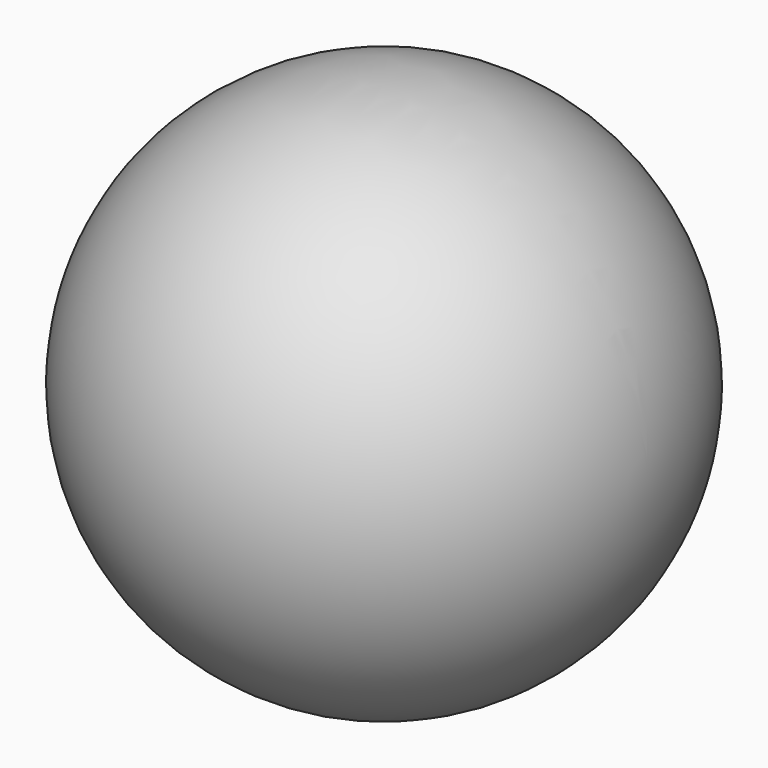
from build123d import *

# Parameters (mm, degrees)
F0_R = 11.165731945


# Not quite as in the source:
# - a feature of the source that left no trace in its solid (it failed there, or was rolled back) is left out


with BuildPart() as f1:
    # F0 (on Front) → F1 (revolve)
    with BuildSketch(Plane.XZ):
        with BuildLine():
            Line((20.728200312, 0), (44.2661586154, 0))
            ThreePointArc((44.2661586154, 0), (0, 44.2661586154), (-44.2661586154, 0))
            Line((-44.2661586154, 0), (7.5460079952, 0))
            ThreePointArc((7.5460079952, 0), (3.7369476756, 32.2853548344), (32.5053808072, 17.1450003982))
            ThreePointArc((32.5053808072, 17.1450003982), (29.2774585899, 6.7448439201), (20.728200312, 0))
        make_face()
        with Locations((-20.7544732839, 15.9418415278)):
            Circle(F0_R, mode=Mode.SUBTRACT)
    revolve(axis=Axis((0, 0, 0), (1, 0, 0)))


solid = f1.part
